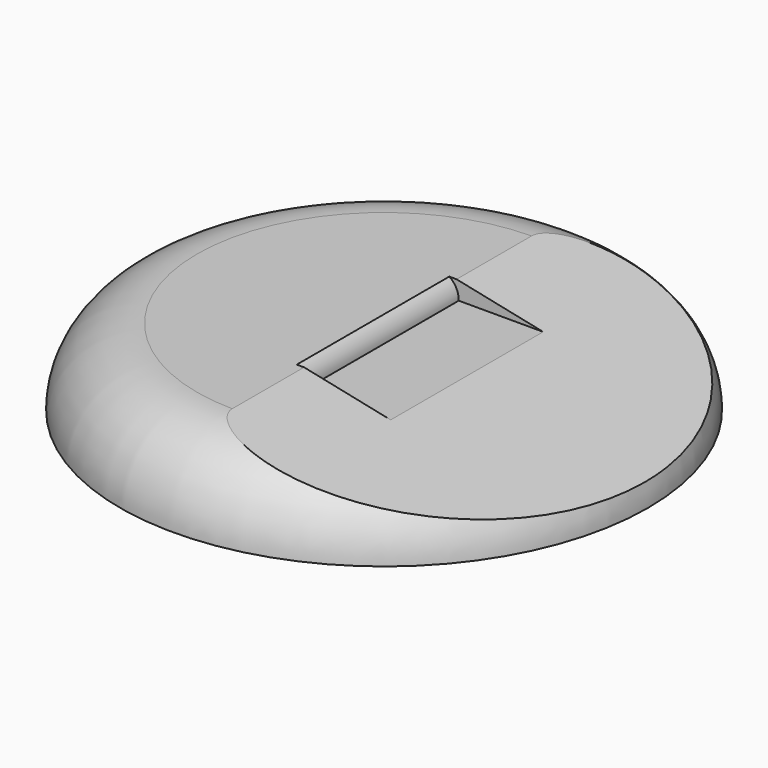
from build123d import *

# Parameters (mm, degrees)
F3_DEPTH      = 37.4664531479
F3_DEPTH_BACK = 37.4664531479
F4_W          = 27.0610069856
F4_H          = 5.9583876282
F5_DEPTH      = 37.4664532479
F6_T1_DEPTH   = 27.0610069856


# Not quite as in the source:
# - a fillet or chamfer that OpenCascade refuses, or shapes differently, is made with other operations: its cross-section is extruded or revolved along the edge and cut away or added


with BuildPart() as f1:
    # F0 (on Front) → F1 (revolve)
    with BuildSketch(Plane.XZ):
        with BuildLine():
            Line((0, 10.9038136992), (0, 0))
            Line((0, 0), (37.4654531479, 0))
            ThreePointArc((37.4654531479, 0), (34.2718000562, 7.7101606075), (26.5616394487, 10.9038136992))
            Line((26.5616394487, 10.9038136992), (0, 10.9038136992))
        make_face()
    revolve(axis=Axis((0, 0, 5.4519068496), (0, 0, 1)))

    # F2 (on Front) → F3 (cut, two sides)
    with BuildSketch(Plane.XZ) as f3_sk:
        Polygon((-10.2507751435, 15.1971811429), (-9.8996739835, 12.9150208086), (41.1855690181, 2.2064307705), (41.1855690181, 15.1971811429), align=None)
    extrude(amount=-F3_DEPTH, mode=Mode.SUBTRACT)
    extrude(f3_sk.sketch, amount=F3_DEPTH_BACK, mode=Mode.SUBTRACT)

    # F4 (on Right) → F5 (cut, through all)
    with BuildSketch(Plane.YZ):
        with Locations((-0.2851500176, 11.3063631579)):
            Rectangle(F4_W, F4_H)
    extrude(amount=F5_DEPTH, mode=Mode.SUBTRACT)

    # F6: fillet of radius 3 on 1 edges, made by hand

    # F6_s2 → F6_t1 (cut)
    with BuildSketch(Plane.XZ.offset(-13.2453534752)):
        with BuildLine():
            ThreePointArc((-2.3845113791, 11.3396775065), (-0.6712164267, 10.2947282416), (0, 8.4034939704))
            Line((0, 8.4034939704), (0, 10.8398314981))
            Line((0, 10.8398314981), (-2.3845113791, 11.3396775065))
        make_face()
    extrude(amount=F6_T1_DEPTH, mode=Mode.SUBTRACT)


solid = f1.part
